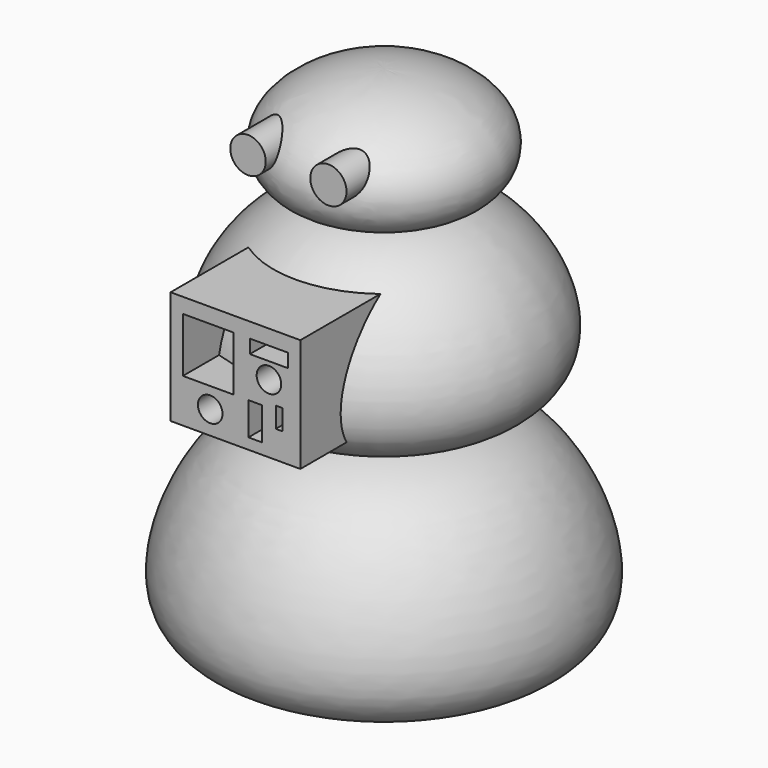
from build123d import *

# Parameters (mm, degrees)
F6_R     = 2.3935238265
F6_R_2   = 2.4454458433
F7_DEPTH = 15.24
F8_R     = 1.6591921449
F8_W     = 1.843548147
F8_H     = 4.4245161116
F8_W_2   = 0.9217732586
F8_H_2   = 2.7653239667
F8_W_3   = 6.8211294711
F8_H_3   = 7.3741972446
F8_R_2   = 1.6591958702
F8_W_4   = 5.1619342994
F8_H_4   = 1.8435493112
F9_DEPTH = 25.4


# Not quite as in the source:
# - the program builds the solid bodies; features that only make, move or delete a surface that nothing else refers to are left out


with BuildPart() as f1:
    # F0 (on Front) → F1 (revolve)
    with BuildSketch(Plane.XZ):
        with BuildLine():
            add(Edge.make_bspline(
                [(0, 29.8654828221), (9.8535054473, 29.2943295833), (20.8212154261, 26.0906949961), (29.5812727595, 0.8606382631), (12.9526836251, -0.6516184138), (0, 0)],
                knots=[0, 0, 0, 0, 0.3341989325, 0.6371981217, 1, 1, 1, 1], degree=3))
            Line((0, 29.8654828221), (0, 0))
        make_face()
    revolve(axis=Axis((0, 0, 4.7932267189), (0, 0, -1)))


with BuildPart() as f3:
    # F2 (on Front) → F3 (revolve)
    with BuildSketch(Plane.XZ):
        with BuildLine():
            add(Edge.make_bspline(
                [(0, 53.8316108286), (6.9928166701, 55.3262349055), (17.4817013102, 50.1793012041), (23.7774783446, 33.6273746897), (12.9733139144, 27.8917889087), (0, 30.2341934294)],
                knots=[0, 0, 0, 0, 0.3362104295, 0.6276333026, 1, 1, 1, 1], degree=3))
            Line((0, 53.8316108286), (0, 30.2341934294))
        make_face()
    revolve(axis=Axis((0, 0, 9.2177409679), (0, 0, -1)))

    # F4 (on Front) → F5 (revolve)
    with BuildSketch(Plane.XZ):
        with BuildLine():
            add(Edge.make_bspline(
                [(0, 68.7643587589), (5.7940934785, 68.9487084746), (15.8255702308, 64.3442509018), (13.700454757, 53.9308476818), (5.0545447701, 53.7009421683), (0, 53.6472573876)],
                knots=[0, 0, 0, 0, 0.3854363626, 0.6434947274, 1, 1, 1, 1], degree=3))
            Line((0, 68.7643587589), (0, 53.6472573876))
        make_face()
    revolve(axis=Axis((0, 0, 15.8545151353), (0, 0, -1)))

    # F6 (on Front) → F7 (join)
    with BuildSketch(Plane.XZ):
        with Locations((-6.1623989604, 62.6971721649)):
            Circle(F6_R)
        with Locations((4.6879197471, 62.6806467772)):
            Circle(F6_R_2)
    extrude(amount=F7_DEPTH)

    # F8 (on Front) → F9 (join)
    with BuildSketch(Plane.XZ):
        Polygon((9.0333875269, 49.7758090496), (-8.4803225473, 49.7758090496), (-8.4803225473, 37.6083850861), (-8.4803225473, 34.4743542373), (9.0333875269, 34.4743542373), align=None)
        with BuildLine():
            ThreePointArc((-5.1619373262, 37.6083850861), (-6.8211294711, 35.9491929412), (-8.4803216159, 37.6083850861))
            ThreePointArc((-8.4803216159, 37.6083850861), (-6.8211294711, 39.2675772309), (-5.1619373262, 37.6083850861))
        make_face(mode=Mode.SUBTRACT)
        with Locations((-3.1340324786, 37.6083850861)):
            Circle(F8_R, mode=Mode.SUBTRACT)
        with Locations((2.9496775242, 38.161450997)):
            Rectangle(F8_W, F8_H, mode=Mode.SUBTRACT)
        with Locations((6.1758875381, 39.544114843)):
            Rectangle(F8_W_2, F8_H_2, mode=Mode.SUBTRACT)
        with Locations((-3.4105647355, 44.0608076751)):
            Rectangle(F8_W_3, F8_H_3, mode=Mode.SUBTRACT)
        with Locations((4.7932254383, 43.6921007931)):
            Circle(F8_R_2, mode=Mode.SUBTRACT)
        with Locations((4.7932254383, 46.8261316419)):
            Rectangle(F8_W_4, F8_H_4, mode=Mode.SUBTRACT)
        with BuildLine():
            ThreePointArc((-5.1619373262, 37.6083850861), (-6.8211294711, 39.2675772309), (-8.4803216159, 37.6083850861))
            ThreePointArc((-8.4803216159, 37.6083850861), (-6.8211294711, 35.9491929412), (-5.1619373262, 37.6083850861))
        make_face()
    extrude(amount=F9_DEPTH)


solid = Compound([f1.part, f3.part])
